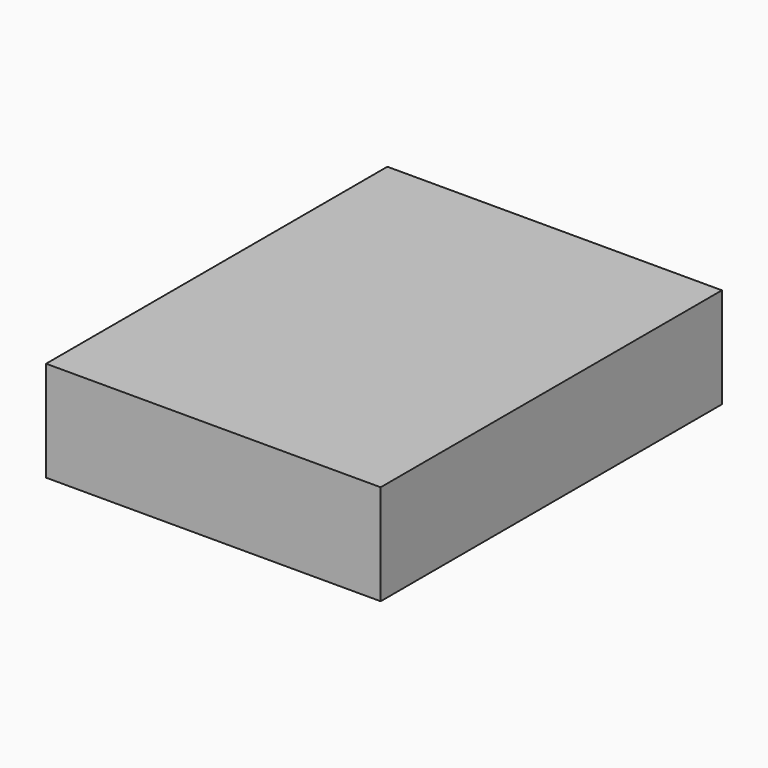
from build123d import *

# Parameters (mm, degrees)
F0_W     = 40
F0_H     = 12
F1_DEPTH = 51


# Not quite as in the source:
# - a feature names something its author has since deleted; it is built from what else it names


with BuildPart() as f1:
    # F0 (on Front) → F1 (new body)
    with BuildSketch(Plane.XZ):
        with Locations((-54.9705135822, 44.4702977538)):
            Rectangle(F0_W, F0_H)
    extrude(amount=F1_DEPTH)


solid = f1.part
